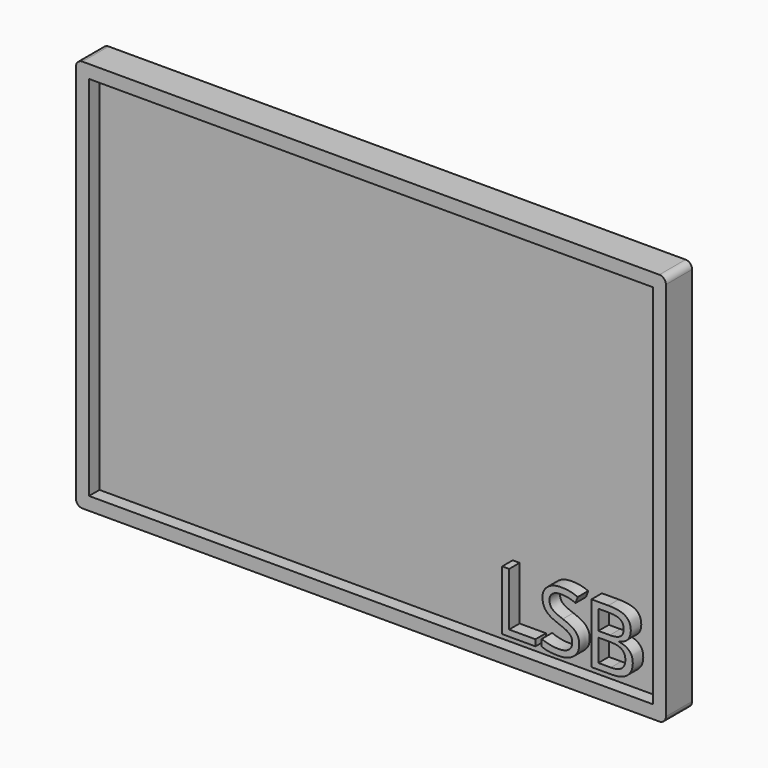
from build123d import *

# Parameters (mm, degrees)
F0_W         = 450
F0_H         = 300
F1_DEPTH     = 25
F2_W         = 430
F2_H         = 280
F3_DEPTH     = 10
F4_W         = 100
F4_H         = 70
F5_DEPTH     = 20
F6_R         = 7.5
F7_DEPTH     = 20
F8_TEXT_SIZE = 63.7248054975
F9_DEPTH     = 10
F10_R        = 5


# Not quite as in the source:
# - Text() gives the source's letters only with a copy of the font that has no kerning and outlines rounded to 1/6400 em; it was checked with that copy


with BuildPart() as f1:
    # F0 (on Front) → F1 (new body)
    with BuildSketch(Plane.XZ):
        Rectangle(F0_W, F0_H)
    extrude(amount=F1_DEPTH)

    # F2 (on face) → F3 (cut)
    with BuildSketch(Plane.XZ.offset(25)):
        Rectangle(F2_W, F2_H)
    extrude(amount=-F3_DEPTH, mode=Mode.SUBTRACT)

    # F4 (on face) → F5 (join)
    with BuildSketch(Plane(origin=(0, 0, 0), x_dir=(-1, 0, 0), z_dir=(0, 1, 0))):
        with Locations((0, -15)):
            Rectangle(F4_W, F4_H)
    extrude(amount=F5_DEPTH)

    # F6 (on face) → F7 (cut)
    with BuildSketch(Plane(origin=(0, 20, 0), x_dir=(-1, 0, 0), z_dir=(0, 1, 0))):
        Circle(F6_R)
    extrude(amount=-F7_DEPTH, mode=Mode.SUBTRACT)

    # F8 (on face) → F9 (join)
    with BuildSketch(Plane.XZ.offset(15)):
        with Locations((93.8952565193, -130.278788507)):
            Text('LSB', F8_TEXT_SIZE, font='Open Sans', text_align=(TextAlign.LEFT, TextAlign.BOTTOM))
    extrude(amount=F9_DEPTH)

    # F10
    f10_edges = [f1.edges().sort_by_distance(p)[0] for p in [
        (-225, -12.5, 150),
        (225, -12.5, 150),
        (225, -12.5, -150),
        (-225, -12.5, -150),
    ]]
    fillet(f10_edges, radius=F10_R)


solid = f1.part
